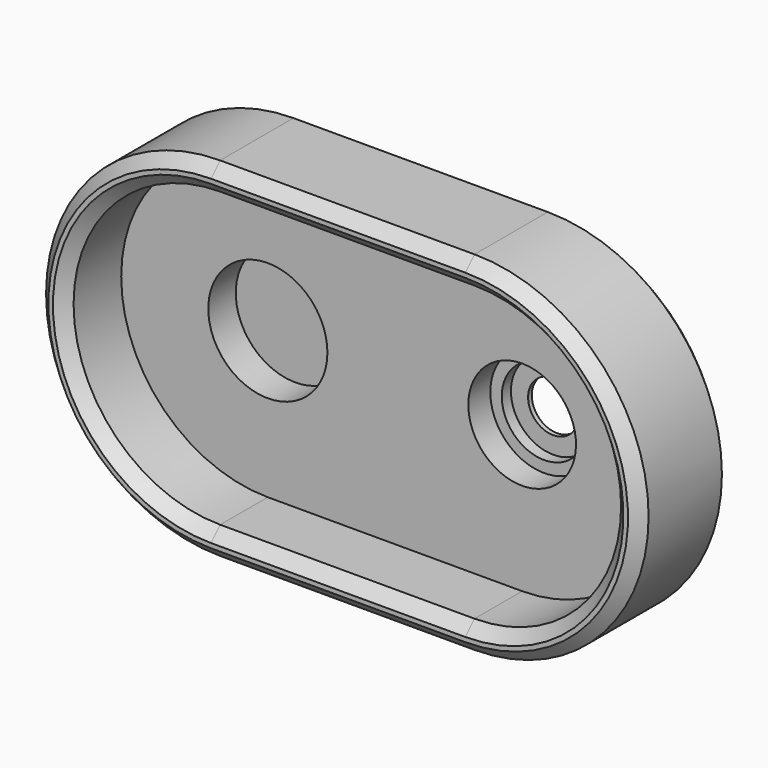
from build123d import *

# Parameters (mm, degrees)
F1_DEPTH = 50
F4_DEPTH = 60
F5_R     = 26
F6_DEPTH = 15
F10_SIZE = 5
F11_SIZE = 5
F12_SIZE = 5


with BuildPart() as f1:
    # F0 (on Front) → F1 (new body)
    with BuildSketch(Plane.XZ):
        with BuildLine():
            Line((111, 76), (0, 76))
            ThreePointArc((0, 76), (-76, 0), (0, -76))
            Line((0, -76), (111, -76))
            ThreePointArc((111, -76), (187, 0), (111, 76))
        make_face()
    extrude(amount=F1_DEPTH)

    # F3 (on offset) + F1_face (on face) → F4 (cut)
    with BuildSketch(Plane.XZ.offset(19)):
        with BuildLine():
            Line((111, 64), (0, 64))
            ThreePointArc((0, 64), (-64, 0), (0, -64))
            Line((0, -64), (111, -64))
            ThreePointArc((111, -64), (175, 0), (111, 64))
        make_face()
    with BuildSketch(Plane(origin=(55.5, -50, 0), x_dir=(1, 0, 0), z_dir=(0, -1, 0))):
        with BuildLine():
            Line((55.5, 76), (-55.5, 76))
            ThreePointArc((-55.5, 76), (-131.5, 0), (-55.5, -76))
            Line((-55.5, -76), (55.5, -76))
            ThreePointArc((55.5, -76), (131.5, 0), (55.5, 76))
        make_face()
    extrude(amount=F4_DEPTH, mode=Mode.SUBTRACT)

    # F5 (on offset) → F6 (cut)
    with BuildSketch(Plane.XZ.offset(19)):
        Circle(F5_R)
    extrude(amount=-F6_DEPTH, mode=Mode.SUBTRACT)

    # F8 (on offset) → F9 (revolve, cut)
    with BuildSketch(Plane.YZ.offset(111)):
        Polygon((0, 0), (0, 11), (-2, 11), (-2, 18.5), (-7, 18.5), (-7, 23.5), (-19, 23.5), (-19, 0), align=None)
    revolve(axis=Axis((111, -9.5, 0), (0, 1, 0)), mode=Mode.SUBTRACT)

    # F10
    f10_edges = [f1.edges().sort_by_distance(p)[0] for p in [
        (55.5, 0, 76),
        (187, 0, 0),
        (-76, 0, 0),
        (55.5, 0, -76),
    ]]
    chamfer(f10_edges, length=F10_SIZE)

    # F11
    f11_edges = [f1.edges().sort_by_distance(p)[0] for p in [
        (55.5, -50, 76),
        (-76, -50, 0),
        (187, -50, 0),
        (55.5, -50, -76),
    ]]
    chamfer(f11_edges, length=F11_SIZE)

    # F12
    f12_edges = [f1.edges().sort_by_distance(p)[0] for p in [
        (55.5, -50, 64),
        (-64, -50, 0),
        (55.5, -50, -64),
        (175, -50, 0),
    ]]
    chamfer(f12_edges, length=F12_SIZE)


solid = f1.part
